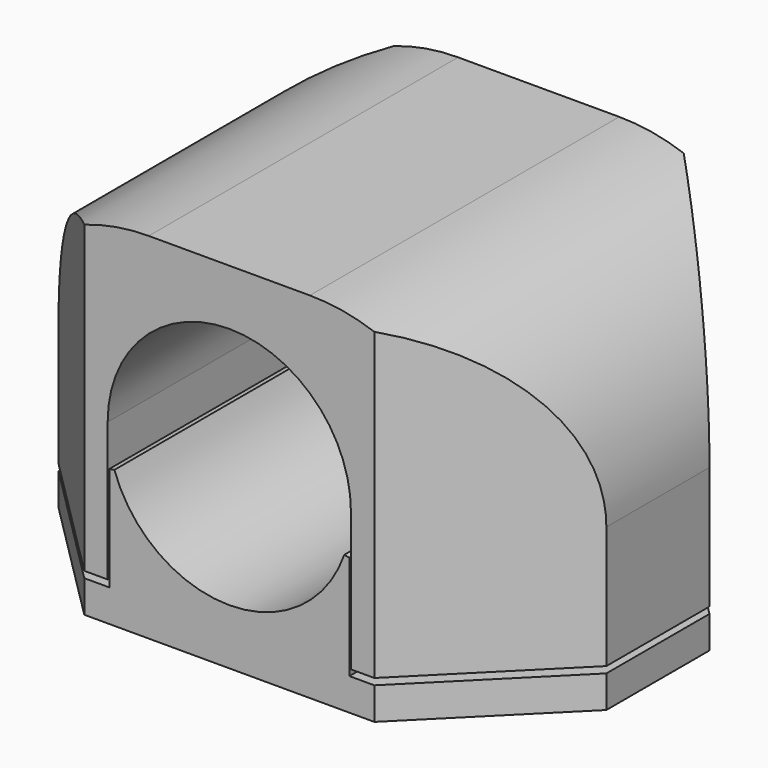
from build123d import *

# Parameters (mm, degrees)
F1_DEPTH    = 24
F2_DEPTH    = 24
F4_DEPTH    = 22.001
F5_R        = 1
F6_DEPTH    = 15
F5_R_2      = 1.4
F7_DEPTH    = 2
F8_T1_DEPTH = 30.6026868141


# Not quite as in the source:
# - a fillet or chamfer that OpenCascade refuses, or shapes differently, is made with other operations: its cross-section is extruded or revolved along the edge and cut away or added


with BuildPart() as f1:
    # F0 (on Front) → F1 (new body)
    with BuildSketch(Plane.XZ):
        with BuildLine():
            Line((7.55, -8.6), (17, -8.6))
            Line((17, -8.6), (17, -1))
            ThreePointArc((17, -1), (13.4852813742, 7.4852813742), (5, 11))
            Line((5, 11), (-5, 11))
            ThreePointArc((-5, 11), (-13.4852813742, 7.4852813742), (-17, -1))
            Line((-17, -1), (-17, -8.6))
            Line((-17, -8.6), (-7.55, -8.6))
            Line((-7.55, -8.6), (-7.55, 0))
            ThreePointArc((-7.55, 0), (0, 7.55), (7.55, 0))
            Line((7.55, 0), (7.55, -8.6))
        make_face()
    extrude(amount=F1_DEPTH)


with BuildPart() as f2:
    # F0 (on Front) → F2 (new body)
    with BuildSketch(Plane.XZ):
        Polygon((-17, -11), (17, -11), (17, -9), (7.45, -9), (-7.45, -9), (-17, -9), align=None)
        with BuildLine():
            Line((-7.45, -9), (7.45, -9))
            Line((7.45, -9), (7.45, -1.2247448714))
            ThreePointArc((7.45, -1.2247448714), (0, -7.55), (-7.45, -1.2247448714))
            Line((-7.45, -1.2247448714), (-7.45, -9))
        make_face()
    extrude(amount=F2_DEPTH)


with BuildPart() as f4_tool:
    # F3 (on face) → F4 (new body, through all)
    with BuildSketch(Plane(origin=(0, 0, -11), x_dir=(1, 0, 0), z_dir=(0, 0, -1))):
        Polygon((-17, 16), (-9, 24), (-17, 24), align=None)
        Polygon((-9, 0), (-17, 8), (-17, 0), align=None)
        Polygon((17, 0), (17, 8), (9, 0), align=None)
        Polygon((17, 24), (9, 24), (17, 16), align=None)
    extrude(amount=-F4_DEPTH)


with BuildPart() as f1_1:
    add(f1.part)

    # F4: cut by f4_tool
    add(f4_tool.part, mode=Mode.SUBTRACT)


with BuildPart() as f2_1:
    add(f2.part)

    # F4: cut by f4_tool
    add(f4_tool.part, mode=Mode.SUBTRACT)


with BuildPart() as f6_tool:
    # F5 (on face) → F6 (new body)
    with BuildSketch(Plane(origin=(0, 0, -11), x_dir=(1, 0, 0), z_dir=(0, 0, -1))):
        with Locations((-12, 12)):
            Circle(F5_R)
        with Locations((12, 12)):
            Circle(F5_R)
    extrude(amount=-F6_DEPTH)


with BuildPart() as f1_2:
    add(f1_1.part)

    # F6: cut by f6_tool
    add(f6_tool.part, mode=Mode.SUBTRACT)


with BuildPart() as f2_2:
    add(f2_1.part)

    # F6: cut by f6_tool
    add(f6_tool.part, mode=Mode.SUBTRACT)

    # F5 (on face) → F7 (cut, through all)
    with BuildSketch(Plane(origin=(0, 0, -11), x_dir=(1, 0, 0), z_dir=(0, 0, -1))):
        with Locations((-12, 12)):
            Circle(F5_R_2)
        with Locations((-12, 12)):
            Circle(F5_R, mode=Mode.SUBTRACT)
        with Locations((12, 12)):
            Circle(F5_R_2)
        with Locations((12, 12)):
            Circle(F5_R, mode=Mode.SUBTRACT)
    extrude(amount=-F7_DEPTH, mode=Mode.SUBTRACT)

    # F8: chamfer of 2 on 2 edges, made by hand

    # F8_s2 → F8_t1 (cut)
    with BuildSketch(Plane.XZ.offset(-3.3013434071)):
        with BuildLine():
            Line((-7.5288861074, -2.5429238838), (-7.0535468383, -2.4627620222))
            Line((-7.0535468383, -2.4627620222), (-7.0157591141, -2.4496437945))
            ThreePointArc((-7.0157591141, -2.4496437945), (-7.2784359572, -1.8505323605), (-7.4105298013, -1.2182561568))
            Line((-7.4105298013, -1.2182561568), (-7.49, -1.2247448714))
            ThreePointArc((-7.49, -1.2247448714), (-7.49, -1.8838343776), (-7.5688861074, -2.5429238838))
            Line((-7.5688861074, -2.5429238838), (-7.5288861074, -2.5429238838))
        make_face()
        with BuildLine():
            Line((7.0535468383, -2.4627620222), (7.5288861074, -2.5429238838))
            Line((7.5288861074, -2.5429238838), (7.5688861074, -2.5429238838))
            ThreePointArc((7.5688861074, -2.5429238838), (7.49, -1.8838343776), (7.49, -1.2247448714))
            Line((7.49, -1.2247448714), (7.4105298013, -1.2182561568))
            ThreePointArc((7.4105298013, -1.2182561568), (7.2784359572, -1.8505323605), (7.0157591141, -2.4496437945))
            Line((7.0157591141, -2.4496437945), (7.0535468383, -2.4627620222))
        make_face()
    extrude(amount=F8_T1_DEPTH, mode=Mode.SUBTRACT)


solid = Compound([f1_2.part, f2_2.part])
